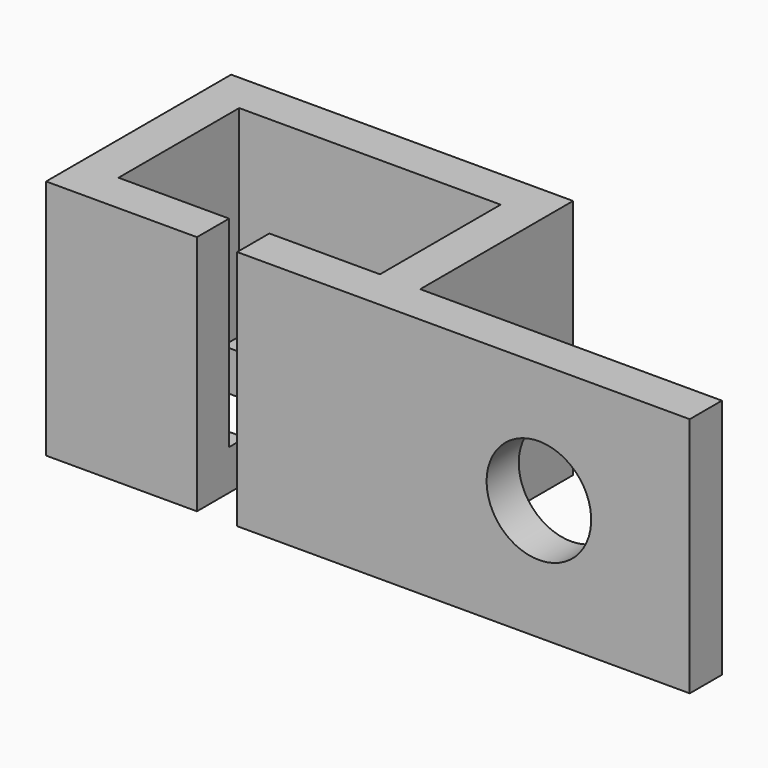
from build123d import *

# Parameters (mm, degrees)
F1_DEPTH     = 10
F2_W         = 5.5
F2_H         = 1
F2_W_2       = 13
F3_DEPTH     = 2
F4_TEXT_SIZE = 3.0279993856
F5_DEPTH     = 0.6
F6_W         = 2
F6_H         = 12
F7_DEPTH     = 15
F8_R         = 2.6
F9_DEPTH     = 2.001


# Not quite as in the source:
# - Text() gives the source's letters only with a copy of the font that has no kerning and outlines rounded to 1/6400 em; it was checked with that copy


with BuildPart() as f1:
    # F0 (on Top) → F1 (new body)
    with BuildSketch(Plane.XY):
        Polygon((-6.5, 3.75), (6.5, 3.75), (6.5, -3.75), (1, -3.75), (1, -5.75), (8.5, -5.75), (8.5, 5.75), (-8.5, 5.75), (-8.5, -5.75), (-1, -5.75), (-1, -3.75), (-6.5, -3.75), align=None)
    extrude(amount=F1_DEPTH)

    # F2 (on face) → F3 (join)
    with BuildSketch(Plane(origin=(0, 0, 0), x_dir=(1, 0, 0), z_dir=(0, 0, -1))):
        with Locations((-3.75, 3.25)):
            Rectangle(F2_W, F2_H)
        Polygon((-1, 5.75), (-8.5, 5.75), (-8.5, -5.75), (8.5, -5.75), (8.5, 5.75), (1, 5.75), (1, 3.75), (6.5, 3.75), (6.5, 2.75), (6.5, -2.75), (6.5, -3.75), (-6.5, -3.75), (-6.5, -2.75), (-6.5, 2.75), (-6.5, 3.75), (-1, 3.75), align=None)
        with Locations((3.75, 3.25)):
            Rectangle(F2_W, F2_H)
        with Locations((0, -3.25)):
            Rectangle(F2_W_2, F2_H)
    extrude(amount=F3_DEPTH)

    # F4 (on face) → F5 (cut)
    with BuildSketch(Plane(origin=(0, 5.75, 0), x_dir=(-1, 0, 0), z_dir=(0, 1, 0))):
        with Locations((-6.2394596171, 7.0113399997)):
            Text('Extruder', F4_TEXT_SIZE, font='Open Sans', text_align=(TextAlign.LEFT, TextAlign.BOTTOM))
        with Locations((-2.3054260403, 2.8932608354)):
            Text('Fan', F4_TEXT_SIZE, font='Open Sans', text_align=(TextAlign.LEFT, TextAlign.BOTTOM))
        with Locations((-6.2394596171, -1.224818329)):
            Text('ON   OFF', F4_TEXT_SIZE, font='Open Sans', text_align=(TextAlign.LEFT, TextAlign.BOTTOM))
    extrude(amount=-F5_DEPTH, mode=Mode.SUBTRACT)

    # F6 (on face) → F7 (join)
    with BuildSketch(Plane.YZ.offset(8.5)):
        with Locations((-4.75, 4)):
            Rectangle(F6_W, F6_H)
    extrude(amount=F7_DEPTH)

    # F8 (on face) → F9 (cut, through all)
    with BuildSketch(Plane(origin=(0, -3.75, 0), x_dir=(-1, 0, 0), z_dir=(0, 1, 0))):
        with Locations((-16, 4)):
            Circle(F8_R)
    extrude(amount=-F9_DEPTH, mode=Mode.SUBTRACT)


solid = f1.part
